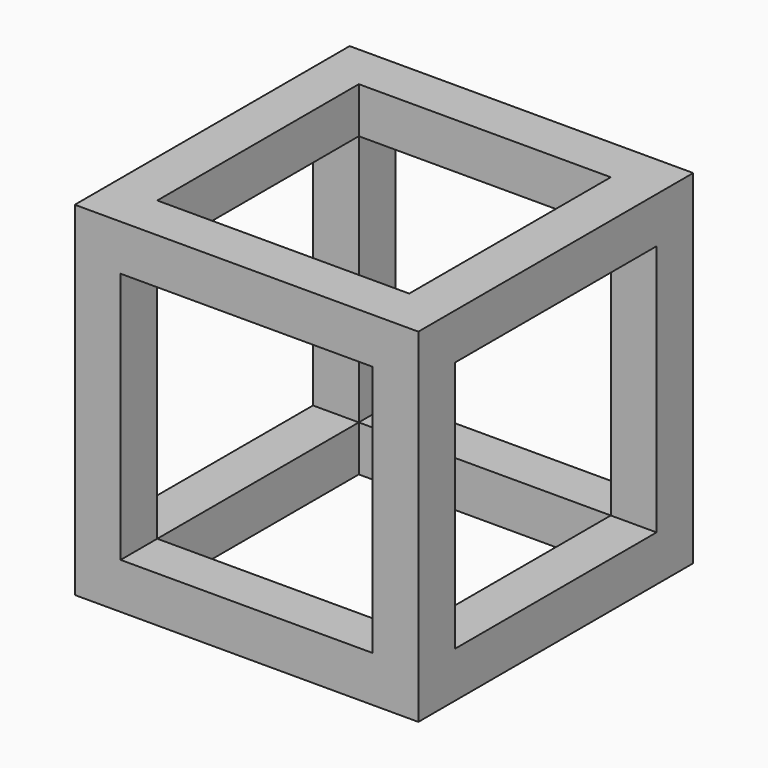
from build123d import *

# Parameters (mm, degrees)
F0_W          = 15
F0_H          = 15
F0_W_2        = 11
F0_H_2        = 11
F1_DEPTH      = 7.5
F1_DEPTH_BACK = 7.5
F2_W          = 11
F2_H          = 11
F3_DEPTH      = 25
F4_W          = 11
F4_H          = 11
F5_DEPTH      = 15.001


# Not quite as in the source:
# - the program builds the solid bodies; features that only make, move or delete a surface that nothing else refers to are left out


with BuildPart() as f1:
    # F0 (on Top) → F1 (new body, two sides)
    with BuildSketch(Plane.XY) as f1_sk:
        Rectangle(F0_W, F0_H)
        Rectangle(F0_W_2, F0_H_2, mode=Mode.SUBTRACT)
    extrude(amount=F1_DEPTH)
    extrude(f1_sk.sketch, amount=-F1_DEPTH_BACK)

    # F2 (on face) → F3 (cut)
    with BuildSketch(Plane.XZ.offset(7.5)):
        Rectangle(F2_W, F2_H)
    extrude(amount=-F3_DEPTH, mode=Mode.SUBTRACT)

    # F4 (on face) → F5 (cut, through all)
    with BuildSketch(Plane.YZ.offset(7.5)):
        Rectangle(F4_W, F4_H)
    extrude(amount=-F5_DEPTH, mode=Mode.SUBTRACT)


solid = f1.part
